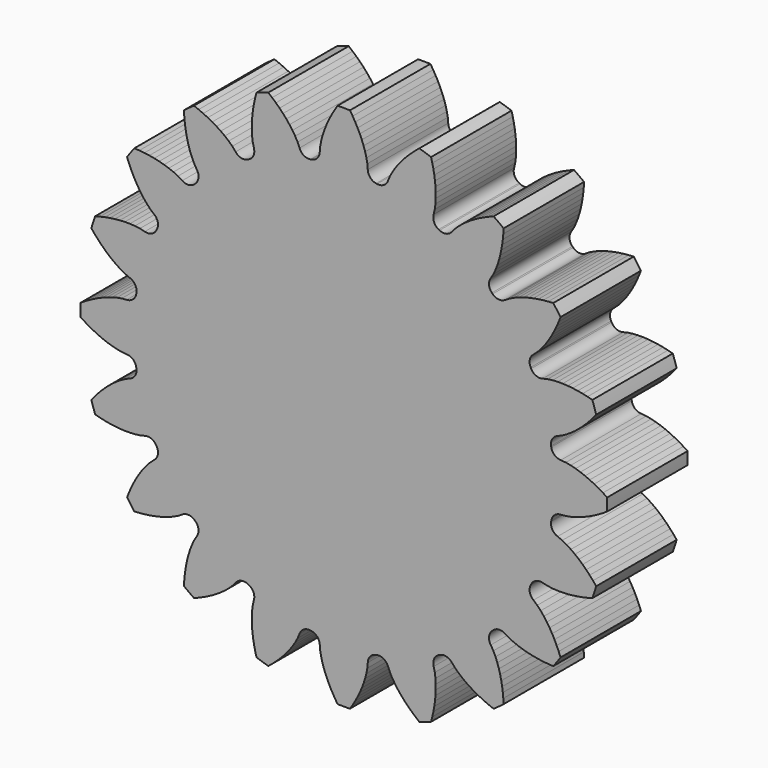
from build123d import *

# Parameters (mm, degrees)
F1_DEPTH = 12.7


# Not quite as in the source:
# - ends of sketch curves that miss each other by under 0.0002 mm in the source are joined


with BuildPart() as f1:
    # F0 (on Front) → F1 (new body)
    with BuildSketch(Plane.XZ):
        with BuildLine():
            ThreePointArc((4.0832280356, 26.2077723122), (3.3388045782, 26.6172297636), (3.030548657, 27.4089367645))
            Line((3.030548657, 27.4089367645), (2.9742892, 28.0403046))
            Line((2.9742892, 28.0403046), (2.8583128, 28.6636968))
            Line((2.8583128, 28.6636968), (2.698623, 29.2774116))
            Line((2.698623, 29.2774116), (2.5031192, 29.880687))
            Line((2.5031192, 29.880687), (2.276729, 30.4730912))
            Line((2.276729, 30.4730912), (2.0230338, 31.0543448))
            Line((2.0230338, 31.0543448), (1.7447514, 31.6242446))
            Line((1.7447514, 31.6242446), (1.444117, 32.1826636))
            Line((1.444117, 32.1826636), (1.1228324, 32.7294748))
            Line((1.1228324, 32.7294748), (0.782701, 33.2648052))
            ThreePointArc((0.782701, 33.2648052), (0, 33.274), (-0.7827007137, 33.264793034))
            Line((-0.7827007137, 33.264793034), (-1.1228324, 32.7294748))
            Line((-1.1228324, 32.7294748), (-1.444117, 32.1826636))
            Line((-1.444117, 32.1826636), (-1.7447514, 31.6242446))
            Line((-1.7447514, 31.6242446), (-2.0230338, 31.0543448))
            Line((-2.0230338, 31.0543448), (-2.276729, 30.4730912))
            Line((-2.276729, 30.4730912), (-2.5031192, 29.880687))
            Line((-2.5031192, 29.880687), (-2.698623, 29.2774116))
            Line((-2.698623, 29.2774116), (-2.8583128, 28.6636968))
            Line((-2.8583128, 28.6636968), (-2.9742892, 28.0403046))
            Line((-2.9742892, 28.0403046), (-3.0305502, 27.4089368))
            ThreePointArc((-3.0305502, 27.4089368), (-3.3388045782, 26.6172297636), (-4.0832280356, 26.2077723122))
            ThreePointArc((-4.0832280356, 26.2077723122), (-4.1492547886, 26.1973969757), (-4.215255651, 26.1868582193))
            ThreePointArc((-4.215255651, 26.1868582193), (-5.0497768191, 26.3462330359), (-5.5876029527, 27.0039305216))
            Line((-5.5876029527, 27.0039305216), (-5.8362088, 27.5870416))
            Line((-5.8362088, 27.5870416), (-6.1391546, 28.1440636))
            Line((-6.1391546, 28.1440636), (-6.480683, 28.6784034))
            Line((-6.480683, 28.6784034), (-6.853047, 29.1917374))
            Line((-6.853047, 29.1917374), (-7.2514206, 29.6851832))
            Line((-7.2514206, 29.6851832), (-7.6722986, 30.1596044))
            Line((-7.6722986, 30.1596044), (-8.1130648, 30.6156106))
            Line((-8.1130648, 30.6156106), (-8.5715602, 31.053786))
            Line((-8.5715602, 31.053786), (-9.046083, 31.4745624))
            Line((-9.046083, 31.4745624), (-9.5350076, 31.8785748))
            ThreePointArc((-9.5350076, 31.8785748), (-10.2822358275, 31.6454531076), (-11.0237774777, 31.3948308822))
            Line((-11.0237774777, 31.3948308822), (-11.181842, 30.780609))
            Line((-11.181842, 30.780609), (-11.3184178, 30.1612808))
            Line((-11.3184178, 30.1612808), (-11.4318034, 29.537279))
            Line((-11.4318034, 29.537279), (-11.5203478, 28.9092894))
            Line((-11.5203478, 28.9092894), (-11.5819936, 28.2780994))
            Line((-11.5819936, 28.2780994), (-11.6142516, 27.644725))
            Line((-11.6142516, 27.644725), (-11.613769, 27.0105378))
            Line((-11.613769, 27.0105378), (-11.5759738, 26.3775444))
            Line((-11.5759738, 26.3775444), (-11.4936524, 25.7488182))
            Line((-11.4936524, 25.7488182), (-11.3520474, 25.1309378))
            ThreePointArc((-11.3520474, 25.1309378), (-11.4005830967, 24.2827403471), (-11.9820288725, 23.6632960769))
            ThreePointArc((-11.9820288725, 23.6632960769), (-12.0416209206, 23.6330126985), (-12.101142224, 23.6025905459))
            ThreePointArc((-12.101142224, 23.6025905459), (-12.9440594727, 23.4962942628), (-13.6587893214, 23.95561113))
            Line((-13.6587893214, 23.95561113), (-14.07541, 24.4333268))
            Line((-14.07541, 24.4333268), (-14.5356834, 24.8694956))
            Line((-14.5356834, 24.8694956), (-15.0255986, 25.2721364))
            Line((-15.0255986, 25.2721364), (-15.5383738, 25.6452878))
            Line((-15.5383738, 25.6452878), (-16.0697164, 25.9914898))
            Line((-16.0697164, 25.9914898), (-16.6166292, 26.3125966))
            Line((-16.6166292, 26.3125966), (-17.1767246, 26.6100814))
            Line((-17.1767246, 26.6100814), (-17.7481992, 26.885138))
            Line((-17.7481992, 26.885138), (-18.329529, 27.1386808))
            Line((-18.329529, 27.1386808), (-18.9193424, 27.3718274))
            ThreePointArc((-18.9193424, 27.3718274), (-19.5579644775, 26.9192329292), (-20.1857582307, 26.451734171))
            Line((-20.1857582307, 26.451734171), (-20.1462894, 25.818719))
            Line((-20.1462894, 25.818719), (-20.084796, 25.1875036))
            Line((-20.084796, 25.1875036), (-19.9998076, 24.559006))
            Line((-19.9998076, 24.559006), (-19.8899526, 23.9343946))
            Line((-19.8899526, 23.9343946), (-19.7535546, 23.315041))
            Line((-19.7535546, 23.315041), (-19.58848, 22.7026978))
            Line((-19.58848, 22.7026978), (-19.3920618, 22.0997018))
            Line((-19.3920618, 22.0997018), (-19.1605154, 21.509355))
            Line((-19.1605154, 21.509355), (-18.887948, 20.936839))
            Line((-18.887948, 20.936839), (-18.5623454, 20.3929742))
            ThreePointArc((-18.5623454, 20.3929742), (-18.3463695047, 19.5712914056), (-18.7079350824, 18.8024738667))
            ThreePointArc((-18.7079350824, 18.8024738667), (-18.7552649089, 18.7552649089), (-18.8024747359, 18.7079359473))
            ThreePointArc((-18.8024747359, 18.7079359473), (-19.5712914056, 18.3463695047), (-20.392976038, 18.562342744))
            Line((-20.392976038, 18.562342744), (-20.936839, 18.887948))
            Line((-20.936839, 18.887948), (-21.509355, 19.1605154))
            Line((-21.509355, 19.1605154), (-22.0997018, 19.3920618))
            Line((-22.0997018, 19.3920618), (-22.7026978, 19.58848))
            Line((-22.7026978, 19.58848), (-23.315041, 19.7535546))
            Line((-23.315041, 19.7535546), (-23.9343946, 19.8899526))
            Line((-23.9343946, 19.8899526), (-24.559006, 19.9998076))
            Line((-24.559006, 19.9998076), (-25.1875036, 20.084796))
            Line((-25.1875036, 20.084796), (-25.818719, 20.1462894))
            Line((-25.818719, 20.1462894), (-26.4517378, 20.185761))
            ThreePointArc((-26.4517378, 20.185761), (-26.9192329292, 19.5579644775), (-27.3718351127, 18.919347731))
            Line((-27.3718351127, 18.919347731), (-27.1386808, 18.329529))
            Line((-27.1386808, 18.329529), (-26.885138, 17.7481992))
            Line((-26.885138, 17.7481992), (-26.6100814, 17.1767246))
            Line((-26.6100814, 17.1767246), (-26.3125966, 16.6166292))
            Line((-26.3125966, 16.6166292), (-25.9914898, 16.0697164))
            Line((-25.9914898, 16.0697164), (-25.6452878, 15.5383738))
            Line((-25.6452878, 15.5383738), (-25.2721364, 15.0255986))
            Line((-25.2721364, 15.0255986), (-24.8694956, 14.5356834))
            Line((-24.8694956, 14.5356834), (-24.4333268, 14.07541))
            Line((-24.4333268, 14.07541), (-23.9556036, 13.6587992))
            ThreePointArc((-23.9556036, 13.6587992), (-23.4962942628, 12.9440594727), (-23.6025869351, 12.1011403728))
            ThreePointArc((-23.6025869351, 12.1011403728), (-23.6330126985, 12.0416209206), (-23.6632847498, 11.9820231369))
            ThreePointArc((-23.6632847498, 11.9820231369), (-24.2827403471, 11.4005830967), (-25.1309357019, 11.3520544013))
            Line((-25.1309357019, 11.3520544013), (-25.7488182, 11.4936524))
            Line((-25.7488182, 11.4936524), (-26.3775444, 11.5759738))
            Line((-26.3775444, 11.5759738), (-27.0105378, 11.613769))
            Line((-27.0105378, 11.613769), (-27.644725, 11.6142516))
            Line((-27.644725, 11.6142516), (-28.2780994, 11.5819936))
            Line((-28.2780994, 11.5819936), (-28.9092894, 11.5203478))
            Line((-28.9092894, 11.5203478), (-29.537279, 11.4318034))
            Line((-29.537279, 11.4318034), (-30.1612808, 11.3184178))
            Line((-30.1612808, 11.3184178), (-30.780609, 11.181842))
            Line((-30.780609, 11.181842), (-31.3948318, 11.0237778))
            ThreePointArc((-31.3948318, 11.0237778), (-31.6454531076, 10.2822358275), (-31.8785629198, 9.5350040466))
            Line((-31.8785629198, 9.5350040466), (-31.4745624, 9.046083))
            Line((-31.4745624, 9.046083), (-31.053786, 8.5715602))
            Line((-31.053786, 8.5715602), (-30.6156106, 8.1130648))
            Line((-30.6156106, 8.1130648), (-30.1596044, 7.6722986))
            Line((-30.1596044, 7.6722986), (-29.6851832, 7.2514206))
            Line((-29.6851832, 7.2514206), (-29.1917374, 6.853047))
            Line((-29.1917374, 6.853047), (-28.6784034, 6.480683))
            Line((-28.6784034, 6.480683), (-28.1440636, 6.1391546))
            Line((-28.1440636, 6.1391546), (-27.5870416, 5.8362088))
            Line((-27.5870416, 5.8362088), (-27.0039338, 5.5875936))
            ThreePointArc((-27.0039338, 5.5875936), (-26.3462330359, 5.0497768191), (-26.1868632921, 4.2152564675))
            ThreePointArc((-26.1868632921, 4.2152564675), (-26.1973969757, 4.1492547886), (-26.207769385, 4.0832275795))
            ThreePointArc((-26.207769385, 4.0832275795), (-26.6172297636, 3.3388045782), (-27.4089367645, 3.030548657))
            Line((-27.4089367645, 3.030548657), (-28.0403046, 2.9742892))
            Line((-28.0403046, 2.9742892), (-28.6636968, 2.8583128))
            Line((-28.6636968, 2.8583128), (-29.2774116, 2.698623))
            Line((-29.2774116, 2.698623), (-29.880687, 2.5031192))
            Line((-29.880687, 2.5031192), (-30.4730912, 2.276729))
            Line((-30.4730912, 2.276729), (-31.0543448, 2.0230338))
            Line((-31.0543448, 2.0230338), (-31.6242446, 1.7447514))
            Line((-31.6242446, 1.7447514), (-32.1826636, 1.444117))
            Line((-32.1826636, 1.444117), (-32.7294748, 1.1228324))
            Line((-32.7294748, 1.1228324), (-33.2648052, 0.782701))
            ThreePointArc((-33.2648052, 0.782701), (-33.274, 0), (-33.264793034, -0.7827007137))
            Line((-33.264793034, -0.7827007137), (-32.7294748, -1.1228324))
            Line((-32.7294748, -1.1228324), (-32.1826636, -1.444117))
            Line((-32.1826636, -1.444117), (-31.6242446, -1.7447514))
            Line((-31.6242446, -1.7447514), (-31.0543448, -2.0230338))
            Line((-31.0543448, -2.0230338), (-30.4730912, -2.276729))
            Line((-30.4730912, -2.276729), (-29.880687, -2.5031192))
            Line((-29.880687, -2.5031192), (-29.2774116, -2.698623))
            Line((-29.2774116, -2.698623), (-28.6636968, -2.8583128))
            Line((-28.6636968, -2.8583128), (-28.0403046, -2.9742892))
            Line((-28.0403046, -2.9742892), (-27.4089368, -3.0305502))
            ThreePointArc((-27.4089368, -3.0305502), (-26.6172297636, -3.3388045782), (-26.2077723122, -4.0832280356))
            ThreePointArc((-26.2077723122, -4.0832280356), (-26.1973969757, -4.1492547886), (-26.1868582193, -4.215255651))
            ThreePointArc((-26.1868582193, -4.215255651), (-26.3462330359, -5.0497768191), (-27.0039305216, -5.5876029527))
            Line((-27.0039305216, -5.5876029527), (-27.5870416, -5.8362088))
            Line((-27.5870416, -5.8362088), (-28.1440636, -6.1391546))
            Line((-28.1440636, -6.1391546), (-28.6784034, -6.480683))
            Line((-28.6784034, -6.480683), (-29.1917374, -6.853047))
            Line((-29.1917374, -6.853047), (-29.6851832, -7.2514206))
            Line((-29.6851832, -7.2514206), (-30.1596044, -7.6722986))
            Line((-30.1596044, -7.6722986), (-30.6156106, -8.1130648))
            Line((-30.6156106, -8.1130648), (-31.053786, -8.5715602))
            Line((-31.053786, -8.5715602), (-31.4745624, -9.046083))
            Line((-31.4745624, -9.046083), (-31.8785748, -9.5350076))
            ThreePointArc((-31.8785748, -9.5350076), (-31.6454531076, -10.2822358275), (-31.3948308822, -11.0237774777))
            Line((-31.3948308822, -11.0237774777), (-30.780609, -11.181842))
            Line((-30.780609, -11.181842), (-30.1612808, -11.3184178))
            Line((-30.1612808, -11.3184178), (-29.537279, -11.4318034))
            Line((-29.537279, -11.4318034), (-28.9092894, -11.5203478))
            Line((-28.9092894, -11.5203478), (-28.2780994, -11.5819936))
            Line((-28.2780994, -11.5819936), (-27.644725, -11.6142516))
            Line((-27.644725, -11.6142516), (-27.0105378, -11.613769))
            Line((-27.0105378, -11.613769), (-26.3775444, -11.5759738))
            Line((-26.3775444, -11.5759738), (-25.7488182, -11.4936524))
            Line((-25.7488182, -11.4936524), (-25.1309378, -11.3520474))
            ThreePointArc((-25.1309378, -11.3520474), (-24.2827403471, -11.4005830967), (-23.6632960769, -11.9820288725))
            ThreePointArc((-23.6632960769, -11.9820288725), (-23.6330126985, -12.0416209206), (-23.6025905459, -12.101142224))
            ThreePointArc((-23.6025905459, -12.101142224), (-23.4962942628, -12.9440594727), (-23.95561113, -13.6587893214))
            Line((-23.95561113, -13.6587893214), (-24.4333268, -14.07541))
            Line((-24.4333268, -14.07541), (-24.8694956, -14.5356834))
            Line((-24.8694956, -14.5356834), (-25.2721364, -15.0255986))
            Line((-25.2721364, -15.0255986), (-25.6452878, -15.5383738))
            Line((-25.6452878, -15.5383738), (-25.9914898, -16.0697164))
            Line((-25.9914898, -16.0697164), (-26.3125966, -16.6166292))
            Line((-26.3125966, -16.6166292), (-26.6100814, -17.1767246))
            Line((-26.6100814, -17.1767246), (-26.885138, -17.7481992))
            Line((-26.885138, -17.7481992), (-27.1386808, -18.329529))
            Line((-27.1386808, -18.329529), (-27.3718274, -18.9193424))
            ThreePointArc((-27.3718274, -18.9193424), (-26.9192329292, -19.5579644775), (-26.451734171, -20.1857582307))
            Line((-26.451734171, -20.1857582307), (-25.818719, -20.1462894))
            Line((-25.818719, -20.1462894), (-25.1875036, -20.084796))
            Line((-25.1875036, -20.084796), (-24.559006, -19.9998076))
            Line((-24.559006, -19.9998076), (-23.9343946, -19.8899526))
            Line((-23.9343946, -19.8899526), (-23.315041, -19.7535546))
            Line((-23.315041, -19.7535546), (-22.7026978, -19.58848))
            Line((-22.7026978, -19.58848), (-22.0997018, -19.3920618))
            Line((-22.0997018, -19.3920618), (-21.509355, -19.1605154))
            Line((-21.509355, -19.1605154), (-20.936839, -18.887948))
            Line((-20.936839, -18.887948), (-20.3929742, -18.5623454))
            ThreePointArc((-20.3929742, -18.5623454), (-19.5712914056, -18.3463695047), (-18.8024738667, -18.7079350824))
            ThreePointArc((-18.8024738667, -18.7079350824), (-18.7552649089, -18.7552649089), (-18.7079359473, -18.8024747359))
            ThreePointArc((-18.7079359473, -18.8024747359), (-18.3463695047, -19.5712914056), (-18.562342744, -20.392976038))
            Line((-18.562342744, -20.392976038), (-18.887948, -20.936839))
            Line((-18.887948, -20.936839), (-19.1605154, -21.509355))
            Line((-19.1605154, -21.509355), (-19.3920618, -22.0997018))
            Line((-19.3920618, -22.0997018), (-19.58848, -22.7026978))
            Line((-19.58848, -22.7026978), (-19.7535546, -23.315041))
            Line((-19.7535546, -23.315041), (-19.8899526, -23.9343946))
            Line((-19.8899526, -23.9343946), (-19.9998076, -24.559006))
            Line((-19.9998076, -24.559006), (-20.084796, -25.1875036))
            Line((-20.084796, -25.1875036), (-20.1462894, -25.818719))
            Line((-20.1462894, -25.818719), (-20.185761, -26.4517378))
            ThreePointArc((-20.185761, -26.4517378), (-19.5579644775, -26.9192329292), (-18.919347731, -27.3718351127))
            Line((-18.919347731, -27.3718351127), (-18.329529, -27.1386808))
            Line((-18.329529, -27.1386808), (-17.7481992, -26.885138))
            Line((-17.7481992, -26.885138), (-17.1767246, -26.6100814))
            Line((-17.1767246, -26.6100814), (-16.6166292, -26.3125966))
            Line((-16.6166292, -26.3125966), (-16.0697164, -25.9914898))
            Line((-16.0697164, -25.9914898), (-15.5383738, -25.6452878))
            Line((-15.5383738, -25.6452878), (-15.0255986, -25.2721364))
            Line((-15.0255986, -25.2721364), (-14.5356834, -24.8694956))
            Line((-14.5356834, -24.8694956), (-14.07541, -24.4333268))
            Line((-14.07541, -24.4333268), (-13.6587992, -23.9556036))
            ThreePointArc((-13.6587992, -23.9556036), (-12.9440594727, -23.4962942628), (-12.1011403728, -23.6025869351))
            ThreePointArc((-12.1011403728, -23.6025869351), (-12.0416209206, -23.6330126985), (-11.9820231369, -23.6632847498))
            ThreePointArc((-11.9820231369, -23.6632847498), (-11.4005830967, -24.2827403471), (-11.3520544013, -25.1309357019))
            Line((-11.3520544013, -25.1309357019), (-11.4936524, -25.7488182))
            Line((-11.4936524, -25.7488182), (-11.5759738, -26.3775444))
            Line((-11.5759738, -26.3775444), (-11.613769, -27.0105378))
            Line((-11.613769, -27.0105378), (-11.6142516, -27.644725))
            Line((-11.6142516, -27.644725), (-11.5819936, -28.2780994))
            Line((-11.5819936, -28.2780994), (-11.5203478, -28.9092894))
            Line((-11.5203478, -28.9092894), (-11.4318034, -29.537279))
            Line((-11.4318034, -29.537279), (-11.3184178, -30.1612808))
            Line((-11.3184178, -30.1612808), (-11.181842, -30.780609))
            Line((-11.181842, -30.780609), (-11.0237778, -31.3948318))
            ThreePointArc((-11.0237778, -31.3948318), (-10.2822358275, -31.6454531076), (-9.5350040466, -31.8785629198))
            Line((-9.5350040466, -31.8785629198), (-9.046083, -31.4745624))
            Line((-9.046083, -31.4745624), (-8.5715602, -31.053786))
            Line((-8.5715602, -31.053786), (-8.1130648, -30.6156106))
            Line((-8.1130648, -30.6156106), (-7.6722986, -30.1596044))
            Line((-7.6722986, -30.1596044), (-7.2514206, -29.6851832))
            Line((-7.2514206, -29.6851832), (-6.853047, -29.1917374))
            Line((-6.853047, -29.1917374), (-6.480683, -28.6784034))
            Line((-6.480683, -28.6784034), (-6.1391546, -28.1440636))
            Line((-6.1391546, -28.1440636), (-5.8362088, -27.5870416))
            Line((-5.8362088, -27.5870416), (-5.5875936, -27.0039338))
            ThreePointArc((-5.5875936, -27.0039338), (-5.0497768191, -26.3462330359), (-4.2152564675, -26.1868632921))
            ThreePointArc((-4.2152564675, -26.1868632921), (-4.1492547886, -26.1973969757), (-4.0832275795, -26.207769385))
            ThreePointArc((-4.0832275795, -26.207769385), (-3.3388045782, -26.6172297636), (-3.030548657, -27.4089367645))
            Line((-3.030548657, -27.4089367645), (-2.9742892, -28.0403046))
            Line((-2.9742892, -28.0403046), (-2.8583128, -28.6636968))
            Line((-2.8583128, -28.6636968), (-2.698623, -29.2774116))
            Line((-2.698623, -29.2774116), (-2.5031192, -29.880687))
            Line((-2.5031192, -29.880687), (-2.276729, -30.4730912))
            Line((-2.276729, -30.4730912), (-2.0230338, -31.0543448))
            Line((-2.0230338, -31.0543448), (-1.7447514, -31.6242446))
            Line((-1.7447514, -31.6242446), (-1.444117, -32.1826636))
            Line((-1.444117, -32.1826636), (-1.1228324, -32.7294748))
            Line((-1.1228324, -32.7294748), (-0.782701, -33.2648052))
            ThreePointArc((-0.782701, -33.2648052), (0, -33.274), (0.7827007137, -33.264793034))
            Line((0.7827007137, -33.264793034), (1.1228324, -32.7294748))
            Line((1.1228324, -32.7294748), (1.444117, -32.1826636))
            Line((1.444117, -32.1826636), (1.7447514, -31.6242446))
            Line((1.7447514, -31.6242446), (2.0230338, -31.0543448))
            Line((2.0230338, -31.0543448), (2.276729, -30.4730912))
            Line((2.276729, -30.4730912), (2.5031192, -29.880687))
            Line((2.5031192, -29.880687), (2.698623, -29.2774116))
            Line((2.698623, -29.2774116), (2.8583128, -28.6636968))
            Line((2.8583128, -28.6636968), (2.9742892, -28.0403046))
            Line((2.9742892, -28.0403046), (3.0305502, -27.4089368))
            ThreePointArc((3.0305502, -27.4089368), (3.3388045782, -26.6172297636), (4.0832280356, -26.2077723122))
            ThreePointArc((4.0832280356, -26.2077723122), (4.1492547886, -26.1973969757), (4.215255651, -26.1868582193))
            ThreePointArc((4.215255651, -26.1868582193), (5.0497768191, -26.3462330359), (5.5876029527, -27.0039305216))
            Line((5.5876029527, -27.0039305216), (5.8362088, -27.5870416))
            Line((5.8362088, -27.5870416), (6.1391546, -28.1440636))
            Line((6.1391546, -28.1440636), (6.480683, -28.6784034))
            Line((6.480683, -28.6784034), (6.853047, -29.1917374))
            Line((6.853047, -29.1917374), (7.2514206, -29.6851832))
            Line((7.2514206, -29.6851832), (7.6722986, -30.1596044))
            Line((7.6722986, -30.1596044), (8.1130648, -30.6156106))
            Line((8.1130648, -30.6156106), (8.5715602, -31.053786))
            Line((8.5715602, -31.053786), (9.046083, -31.4745624))
            Line((9.046083, -31.4745624), (9.5350076, -31.8785748))
            ThreePointArc((9.5350076, -31.8785748), (10.2822358275, -31.6454531076), (11.0237774777, -31.3948308822))
            Line((11.0237774777, -31.3948308822), (11.181842, -30.780609))
            Line((11.181842, -30.780609), (11.3184178, -30.1612808))
            Line((11.3184178, -30.1612808), (11.4318034, -29.537279))
            Line((11.4318034, -29.537279), (11.5203478, -28.9092894))
            Line((11.5203478, -28.9092894), (11.5819936, -28.2780994))
            Line((11.5819936, -28.2780994), (11.6142516, -27.644725))
            Line((11.6142516, -27.644725), (11.613769, -27.0105378))
            Line((11.613769, -27.0105378), (11.5759738, -26.3775444))
            Line((11.5759738, -26.3775444), (11.4936524, -25.7488182))
            Line((11.4936524, -25.7488182), (11.3520474, -25.1309378))
            ThreePointArc((11.3520474, -25.1309378), (11.4005830967, -24.2827403471), (11.9820288725, -23.6632960769))
            ThreePointArc((11.9820288725, -23.6632960769), (12.0416209206, -23.6330126985), (12.101142224, -23.6025905459))
            ThreePointArc((12.101142224, -23.6025905459), (12.9440594727, -23.4962942628), (13.6587893214, -23.95561113))
            Line((13.6587893214, -23.95561113), (14.07541, -24.4333268))
            Line((14.07541, -24.4333268), (14.5356834, -24.8694956))
            Line((14.5356834, -24.8694956), (15.0255986, -25.2721364))
            Line((15.0255986, -25.2721364), (15.5383738, -25.6452878))
            Line((15.5383738, -25.6452878), (16.0697164, -25.9914898))
            Line((16.0697164, -25.9914898), (16.6166292, -26.3125966))
            Line((16.6166292, -26.3125966), (17.1767246, -26.6100814))
            Line((17.1767246, -26.6100814), (17.7481992, -26.885138))
            Line((17.7481992, -26.885138), (18.329529, -27.1386808))
            Line((18.329529, -27.1386808), (18.9193424, -27.3718274))
            ThreePointArc((18.9193424, -27.3718274), (19.5579644775, -26.9192329292), (20.1857582307, -26.451734171))
            Line((20.1857582307, -26.451734171), (20.1462894, -25.818719))
            Line((20.1462894, -25.818719), (20.084796, -25.1875036))
            Line((20.084796, -25.1875036), (19.9998076, -24.559006))
            Line((19.9998076, -24.559006), (19.8899526, -23.9343946))
            Line((19.8899526, -23.9343946), (19.7535546, -23.315041))
            Line((19.7535546, -23.315041), (19.58848, -22.7026978))
            Line((19.58848, -22.7026978), (19.3920618, -22.0997018))
            Line((19.3920618, -22.0997018), (19.1605154, -21.509355))
            Line((19.1605154, -21.509355), (18.887948, -20.936839))
            Line((18.887948, -20.936839), (18.5623454, -20.3929742))
            ThreePointArc((18.5623454, -20.3929742), (18.3463695047, -19.5712914056), (18.7079350824, -18.8024738667))
            ThreePointArc((18.7079350824, -18.8024738667), (18.7552649089, -18.7552649089), (18.8024747359, -18.7079359473))
            ThreePointArc((18.8024747359, -18.7079359473), (19.5712914056, -18.3463695047), (20.392976038, -18.562342744))
            Line((20.392976038, -18.562342744), (20.936839, -18.887948))
            Line((20.936839, -18.887948), (21.509355, -19.1605154))
            Line((21.509355, -19.1605154), (22.0997018, -19.3920618))
            Line((22.0997018, -19.3920618), (22.7026978, -19.58848))
            Line((22.7026978, -19.58848), (23.315041, -19.7535546))
            Line((23.315041, -19.7535546), (23.9343946, -19.8899526))
            Line((23.9343946, -19.8899526), (24.559006, -19.9998076))
            Line((24.559006, -19.9998076), (25.1875036, -20.084796))
            Line((25.1875036, -20.084796), (25.818719, -20.1462894))
            Line((25.818719, -20.1462894), (26.4517378, -20.185761))
            ThreePointArc((26.4517378, -20.185761), (26.9192329292, -19.5579644775), (27.3718351127, -18.919347731))
            Line((27.3718351127, -18.919347731), (27.1386808, -18.329529))
            Line((27.1386808, -18.329529), (26.885138, -17.7481992))
            Line((26.885138, -17.7481992), (26.6100814, -17.1767246))
            Line((26.6100814, -17.1767246), (26.3125966, -16.6166292))
            Line((26.3125966, -16.6166292), (25.9914898, -16.0697164))
            Line((25.9914898, -16.0697164), (25.6452878, -15.5383738))
            Line((25.6452878, -15.5383738), (25.2721364, -15.0255986))
            Line((25.2721364, -15.0255986), (24.8694956, -14.5356834))
            Line((24.8694956, -14.5356834), (24.4333268, -14.07541))
            Line((24.4333268, -14.07541), (23.9556036, -13.6587992))
            ThreePointArc((23.9556036, -13.6587992), (23.4962942628, -12.9440594727), (23.6025869351, -12.1011403728))
            ThreePointArc((23.6025869351, -12.1011403728), (23.6330126985, -12.0416209206), (23.6632847498, -11.9820231369))
            ThreePointArc((23.6632847498, -11.9820231369), (24.2827403471, -11.4005830967), (25.1309357019, -11.3520544013))
            Line((25.1309357019, -11.3520544013), (25.7488182, -11.4936524))
            Line((25.7488182, -11.4936524), (26.3775444, -11.5759738))
            Line((26.3775444, -11.5759738), (27.0105378, -11.613769))
            Line((27.0105378, -11.613769), (27.644725, -11.6142516))
            Line((27.644725, -11.6142516), (28.2780994, -11.5819936))
            Line((28.2780994, -11.5819936), (28.9092894, -11.5203478))
            Line((28.9092894, -11.5203478), (29.537279, -11.4318034))
            Line((29.537279, -11.4318034), (30.1612808, -11.3184178))
            Line((30.1612808, -11.3184178), (30.780609, -11.181842))
            Line((30.780609, -11.181842), (31.3948318, -11.0237778))
            ThreePointArc((31.3948318, -11.0237778), (31.6454531076, -10.2822358275), (31.8785629198, -9.5350040466))
            Line((31.8785629198, -9.5350040466), (31.4745624, -9.046083))
            Line((31.4745624, -9.046083), (31.053786, -8.5715602))
            Line((31.053786, -8.5715602), (30.6156106, -8.1130648))
            Line((30.6156106, -8.1130648), (30.1596044, -7.6722986))
            Line((30.1596044, -7.6722986), (29.6851832, -7.2514206))
            Line((29.6851832, -7.2514206), (29.1917374, -6.853047))
            Line((29.1917374, -6.853047), (28.6784034, -6.480683))
            Line((28.6784034, -6.480683), (28.1440636, -6.1391546))
            Line((28.1440636, -6.1391546), (27.5870416, -5.8362088))
            Line((27.5870416, -5.8362088), (27.0039338, -5.5875936))
            ThreePointArc((27.0039338, -5.5875936), (26.3462330359, -5.0497768191), (26.1868632921, -4.2152564675))
            ThreePointArc((26.1868632921, -4.2152564675), (26.1973969757, -4.1492547886), (26.207769385, -4.0832275795))
            ThreePointArc((26.207769385, -4.0832275795), (26.6172297636, -3.3388045782), (27.4089367645, -3.030548657))
            Line((27.4089367645, -3.030548657), (28.0403046, -2.9742892))
            Line((28.0403046, -2.9742892), (28.6636968, -2.8583128))
            Line((28.6636968, -2.8583128), (29.2774116, -2.698623))
            Line((29.2774116, -2.698623), (29.880687, -2.5031192))
            Line((29.880687, -2.5031192), (30.4730912, -2.276729))
            Line((30.4730912, -2.276729), (31.0543448, -2.0230338))
            Line((31.0543448, -2.0230338), (31.6242446, -1.7447514))
            Line((31.6242446, -1.7447514), (32.1826636, -1.444117))
            Line((32.1826636, -1.444117), (32.7294748, -1.1228324))
            Line((32.7294748, -1.1228324), (33.2648052, -0.782701))
            ThreePointArc((33.2648052, -0.782701), (33.274, 0), (33.264793034, 0.7827007137))
            Line((33.264793034, 0.7827007137), (32.7294748, 1.1228324))
            Line((32.7294748, 1.1228324), (32.1826636, 1.444117))
            Line((32.1826636, 1.444117), (31.6242446, 1.7447514))
            Line((31.6242446, 1.7447514), (31.0543448, 2.0230338))
            Line((31.0543448, 2.0230338), (30.4730912, 2.276729))
            Line((30.4730912, 2.276729), (29.880687, 2.5031192))
            Line((29.880687, 2.5031192), (29.2774116, 2.698623))
            Line((29.2774116, 2.698623), (28.6636968, 2.8583128))
            Line((28.6636968, 2.8583128), (28.0403046, 2.9742892))
            Line((28.0403046, 2.9742892), (27.4089368, 3.0305502))
            ThreePointArc((27.4089368, 3.0305502), (26.6172297636, 3.3388045782), (26.2077723122, 4.0832280356))
            ThreePointArc((26.2077723122, 4.0832280356), (26.1973969757, 4.1492547886), (26.1868582193, 4.215255651))
            ThreePointArc((26.1868582193, 4.215255651), (26.3462330359, 5.0497768191), (27.0039305216, 5.5876029527))
            Line((27.0039305216, 5.5876029527), (27.5870416, 5.8362088))
            Line((27.5870416, 5.8362088), (28.1440636, 6.1391546))
            Line((28.1440636, 6.1391546), (28.6784034, 6.480683))
            Line((28.6784034, 6.480683), (29.1917374, 6.853047))
            Line((29.1917374, 6.853047), (29.6851832, 7.2514206))
            Line((29.6851832, 7.2514206), (30.1596044, 7.6722986))
            Line((30.1596044, 7.6722986), (30.6156106, 8.1130648))
            Line((30.6156106, 8.1130648), (31.053786, 8.5715602))
            Line((31.053786, 8.5715602), (31.4745624, 9.046083))
            Line((31.4745624, 9.046083), (31.8785748, 9.5350076))
            ThreePointArc((31.8785748, 9.5350076), (31.6454531076, 10.2822358275), (31.3948308822, 11.0237774777))
            Line((31.3948308822, 11.0237774777), (30.780609, 11.181842))
            Line((30.780609, 11.181842), (30.1612808, 11.3184178))
            Line((30.1612808, 11.3184178), (29.537279, 11.4318034))
            Line((29.537279, 11.4318034), (28.9092894, 11.5203478))
            Line((28.9092894, 11.5203478), (28.2780994, 11.5819936))
            Line((28.2780994, 11.5819936), (27.644725, 11.6142516))
            Line((27.644725, 11.6142516), (27.0105378, 11.613769))
            Line((27.0105378, 11.613769), (26.3775444, 11.5759738))
            Line((26.3775444, 11.5759738), (25.7488182, 11.4936524))
            Line((25.7488182, 11.4936524), (25.1309378, 11.3520474))
            ThreePointArc((25.1309378, 11.3520474), (24.2827403471, 11.4005830967), (23.6632960769, 11.9820288725))
            ThreePointArc((23.6632960769, 11.9820288725), (23.6330126985, 12.0416209206), (23.6025905459, 12.101142224))
            ThreePointArc((23.6025905459, 12.101142224), (23.4962942628, 12.9440594727), (23.95561113, 13.6587893214))
            Line((23.95561113, 13.6587893214), (24.4333268, 14.07541))
            Line((24.4333268, 14.07541), (24.8694956, 14.5356834))
            Line((24.8694956, 14.5356834), (25.2721364, 15.0255986))
            Line((25.2721364, 15.0255986), (25.6452878, 15.5383738))
            Line((25.6452878, 15.5383738), (25.9914898, 16.0697164))
            Line((25.9914898, 16.0697164), (26.3125966, 16.6166292))
            Line((26.3125966, 16.6166292), (26.6100814, 17.1767246))
            Line((26.6100814, 17.1767246), (26.885138, 17.7481992))
            Line((26.885138, 17.7481992), (27.1386808, 18.329529))
            Line((27.1386808, 18.329529), (27.3718274, 18.9193424))
            ThreePointArc((27.3718274, 18.9193424), (26.9192329292, 19.5579644775), (26.451734171, 20.1857582307))
            Line((26.451734171, 20.1857582307), (25.818719, 20.1462894))
            Line((25.818719, 20.1462894), (25.1875036, 20.084796))
            Line((25.1875036, 20.084796), (24.559006, 19.9998076))
            Line((24.559006, 19.9998076), (23.9343946, 19.8899526))
            Line((23.9343946, 19.8899526), (23.315041, 19.7535546))
            Line((23.315041, 19.7535546), (22.7026978, 19.58848))
            Line((22.7026978, 19.58848), (22.0997018, 19.3920618))
            Line((22.0997018, 19.3920618), (21.509355, 19.1605154))
            Line((21.509355, 19.1605154), (20.936839, 18.887948))
            Line((20.936839, 18.887948), (20.3929742, 18.5623454))
            ThreePointArc((20.3929742, 18.5623454), (19.5712914056, 18.3463695047), (18.8024738667, 18.7079350824))
            ThreePointArc((18.8024738667, 18.7079350824), (18.7552649089, 18.7552649089), (18.7079359473, 18.8024747359))
            ThreePointArc((18.7079359473, 18.8024747359), (18.3463695047, 19.5712914056), (18.562342744, 20.392976038))
            Line((18.562342744, 20.392976038), (18.887948, 20.936839))
            Line((18.887948, 20.936839), (19.1605154, 21.509355))
            Line((19.1605154, 21.509355), (19.3920618, 22.0997018))
            Line((19.3920618, 22.0997018), (19.58848, 22.7026978))
            Line((19.58848, 22.7026978), (19.7535546, 23.315041))
            Line((19.7535546, 23.315041), (19.8899526, 23.9343946))
            Line((19.8899526, 23.9343946), (19.9998076, 24.559006))
            Line((19.9998076, 24.559006), (20.084796, 25.1875036))
            Line((20.084796, 25.1875036), (20.1462894, 25.818719))
            Line((20.1462894, 25.818719), (20.185761, 26.4517378))
            ThreePointArc((20.185761, 26.4517378), (19.5579644775, 26.9192329292), (18.919347731, 27.3718351127))
            Line((18.919347731, 27.3718351127), (18.329529, 27.1386808))
            Line((18.329529, 27.1386808), (17.7481992, 26.885138))
            Line((17.7481992, 26.885138), (17.1767246, 26.6100814))
            Line((17.1767246, 26.6100814), (16.6166292, 26.3125966))
            Line((16.6166292, 26.3125966), (16.0697164, 25.9914898))
            Line((16.0697164, 25.9914898), (15.5383738, 25.6452878))
            Line((15.5383738, 25.6452878), (15.0255986, 25.2721364))
            Line((15.0255986, 25.2721364), (14.5356834, 24.8694956))
            Line((14.5356834, 24.8694956), (14.07541, 24.4333268))
            Line((14.07541, 24.4333268), (13.6587992, 23.9556036))
            ThreePointArc((13.6587992, 23.9556036), (12.9440594727, 23.4962942628), (12.1011403728, 23.6025869351))
            ThreePointArc((12.1011403728, 23.6025869351), (12.0416209206, 23.6330126985), (11.9820231369, 23.6632847498))
            ThreePointArc((11.9820231369, 23.6632847498), (11.4005830967, 24.2827403471), (11.3520544013, 25.1309357019))
            Line((11.3520544013, 25.1309357019), (11.4936524, 25.7488182))
            Line((11.4936524, 25.7488182), (11.5759738, 26.3775444))
            Line((11.5759738, 26.3775444), (11.613769, 27.0105378))
            Line((11.613769, 27.0105378), (11.6142516, 27.644725))
            Line((11.6142516, 27.644725), (11.5819936, 28.2780994))
            Line((11.5819936, 28.2780994), (11.5203478, 28.9092894))
            Line((11.5203478, 28.9092894), (11.4318034, 29.537279))
            Line((11.4318034, 29.537279), (11.3184178, 30.1612808))
            Line((11.3184178, 30.1612808), (11.181842, 30.780609))
            Line((11.181842, 30.780609), (11.0237778, 31.3948318))
            ThreePointArc((11.0237778, 31.3948318), (10.2822358275, 31.6454531076), (9.5350040466, 31.8785629198))
            Line((9.5350040466, 31.8785629198), (9.046083, 31.4745624))
            Line((9.046083, 31.4745624), (8.5715602, 31.053786))
            Line((8.5715602, 31.053786), (8.1130648, 30.6156106))
            Line((8.1130648, 30.6156106), (7.6722986, 30.1596044))
            Line((7.6722986, 30.1596044), (7.2514206, 29.6851832))
            Line((7.2514206, 29.6851832), (6.853047, 29.1917374))
            Line((6.853047, 29.1917374), (6.480683, 28.6784034))
            Line((6.480683, 28.6784034), (6.1391546, 28.1440636))
            Line((6.1391546, 28.1440636), (5.8362088, 27.5870416))
            Line((5.8362088, 27.5870416), (5.5875936, 27.0039338))
            ThreePointArc((5.5875936, 27.0039338), (5.0497768191, 26.3462330359), (4.2152564675, 26.1868632921))
            ThreePointArc((4.2152564675, 26.1868632921), (4.1492547886, 26.1973969757), (4.0832280356, 26.2077723122))
        make_face()
    extrude(amount=F1_DEPTH)


solid = f1.part
